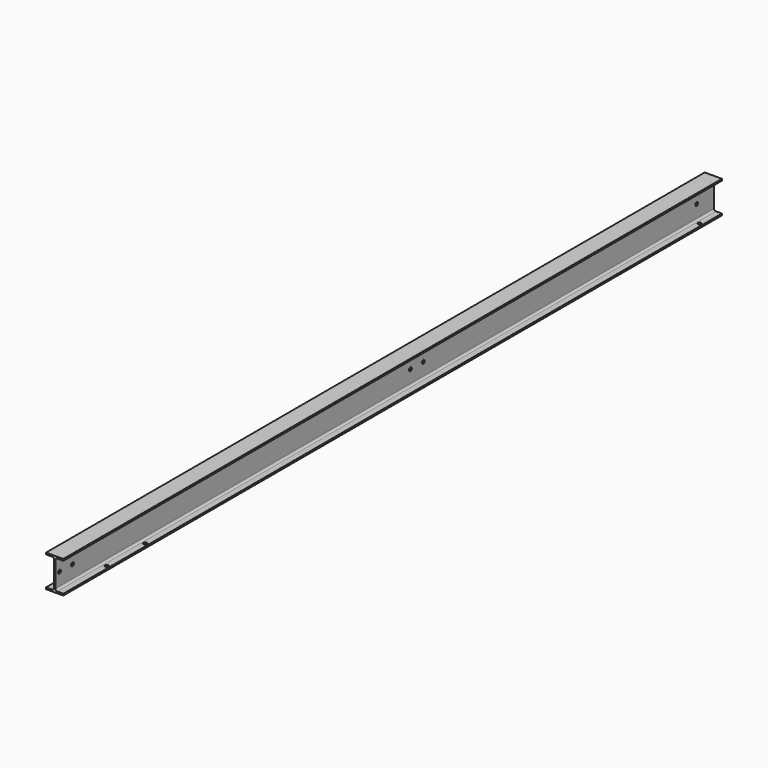
from build123d import *

# Parameters (mm, degrees)
F1_DEPTH      = 300
F1_DEPTH_BACK = 2760
F2_R          = 6.5
F3_DEPTH      = 6.3
F4_R          = 6.5
F5_DEPTH      = 34.201


# Not quite as in the source:
# - a feature names something its author has since deleted; it is built from what else it names


with BuildPart() as f1:
    # F0 (on Front) → F1 (new body, two sides)
    with BuildSketch(Plane.XZ) as f1_sk:
        with BuildLine():
            Line((-32, 6.3), (-32, 0))
            Line((-32, 0), (32, 0))
            Line((32, 0), (32, 6.3))
            Line((32, 6.3), (9.2, 6.3))
            ThreePointArc((9.2, 6.3), (4.2502525317, 8.3502525317), (2.2, 13.3))
            Line((2.2, 13.3), (2.2, 106.7))
            ThreePointArc((2.2, 106.7), (4.2502525317, 111.6497474683), (9.2, 113.7))
            Line((9.2, 113.7), (32, 113.7))
            Line((32, 113.7), (32, 120))
            Line((32, 120), (-32, 120))
            Line((-32, 120), (-32, 113.7))
            Line((-32, 113.7), (-9.2, 113.7))
            ThreePointArc((-9.2, 113.7), (-4.2502525317, 111.6497474683), (-2.2, 106.7))
            Line((-2.2, 106.7), (-2.2, 13.3))
            ThreePointArc((-2.2, 13.3), (-4.2502525317, 8.3502525317), (-9.2, 6.3))
            Line((-9.2, 6.3), (-32, 6.3))
        make_face()
    extrude(amount=F1_DEPTH)
    extrude(f1_sk.sketch, amount=-F1_DEPTH_BACK)

    # F2 (on face) → F3 (cut, through all)
    with BuildSketch(Plane(origin=(0, 0, 0), x_dir=(1, 0, 0), z_dir=(0, 0, -1))):
        with Locations((21, 85)):
            Circle(F2_R)
        with Locations((-21, 85)):
            Circle(F2_R)
        with Locations((-21, -95)):
            Circle(F2_R)
        with Locations((21, -95)):
            Circle(F2_R)
        with Locations((-21, -2670)):
            Circle(F2_R)
        with Locations((21, -2670)):
            Circle(F2_R)
    extrude(amount=-F3_DEPTH, mode=Mode.SUBTRACT)

    # F4 (on face) → F5 (cut, through all)
    with BuildSketch(Plane.YZ.offset(2.2)):
        with Locations((2680, 60)):
            Circle(F4_R)
        with Locations((-280, 60)):
            Circle(F4_R)
        with Locations((-220, 60)):
            Circle(F4_R)
        with Locations((1350, 60)):
            Circle(F4_R)
        with Locations((1410, 60)):
            Circle(F4_R)
    extrude(amount=-F5_DEPTH, mode=Mode.SUBTRACT)


solid = f1.part
